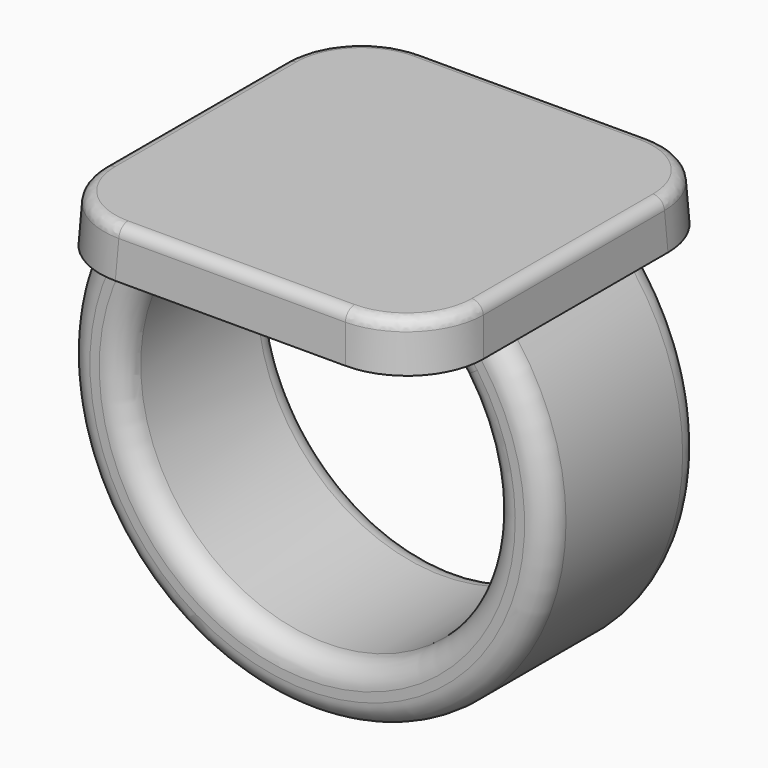
from build123d import *

# Parameters (mm, degrees)
F0_W          = 25.4
F0_H          = 25.4
F1_DEPTH      = 3.175
F1_TAPER      = 3
F3_W          = 5.08
F3_H          = 12.7
F6_DEPTH      = 6.35
F6_DEPTH_BACK = 6.35
F7_R          = 5.08
F8_R          = 1.524
F9_R          = 0.762


with BuildPart() as f1:
    # F0 (on Top) → F1 (new body)
    with BuildSketch(Plane.XY):
        Rectangle(F0_W, F0_H)
    extrude(amount=F1_DEPTH, taper=F1_TAPER)

    # F4: sweep along a path in F2
    with BuildLine(Plane.XZ) as f4_path:
        ThreePointArc((-10.16, 0), (0, -23.5582897328), (10.16, 0))
    # F3 (on face) → F4 (sweep)
    with BuildSketch(Plane(origin=(0, 0, 0), x_dir=(1, 0, 0), z_dir=(0, 0, -1))):
        with Locations((-10.16, 0)):
            Rectangle(F3_W, F3_H)
    sweep(path=f4_path.line)

    # F5 (on Front) → F6 (join, two sides)
    with BuildSketch(Plane.XZ) as f6_sk:
        with BuildLine():
            Line((10.0130578512, -2.535746045), (10.16, 0))
            Line((10.16, 0), (7.62, 0))
            ThreePointArc((7.62, 0), (8.9072265211, -1.1822790439), (10.0130578512, -2.535746045))
        make_face()
    extrude(amount=F6_DEPTH)
    extrude(f6_sk.sketch, amount=-F6_DEPTH_BACK)

    # F7
    f7_edges = [f1.edges().sort_by_distance(p)[0] for p in [
        (-12.616803, -12.616803, 1.5875),
        (-12.616803, 12.616803, 1.5875),
        (12.616803, -12.616803, 1.5875),
        (12.616803, 12.616803, 1.5875),
    ]]
    fillet(f7_edges, radius=F7_R)

    # F8
    f8_edges = [f1.edges().sort_by_distance(p)[0] for p in [
        (-1.743325, -6.35, -21.711017),
        (8.907227, -6.35, -1.182279),
        (-1.743325, 6.35, -21.711017),
        (0, -6.35, -25.501344),
        (0, 6.35, -25.501344),
        (8.907227, 6.35, -1.182279),
    ]]
    fillet(f8_edges, radius=F8_R)

    # F9
    f9_edges = [f1.edges().sort_by_distance(p)[0] for p in [
        (12.533605, 0, 3.175),
        (11.048589, -11.048589, 3.175),
        (11.048589, 11.048589, 3.175),
        (0, -12.533605, 3.175),
        (0, 12.533605, 3.175),
        (-11.048589, -11.048589, 3.175),
        (-11.048589, 11.048589, 3.175),
        (-12.533605, 0, 3.175),
    ]]
    fillet(f9_edges, radius=F9_R)


solid = f1.part
